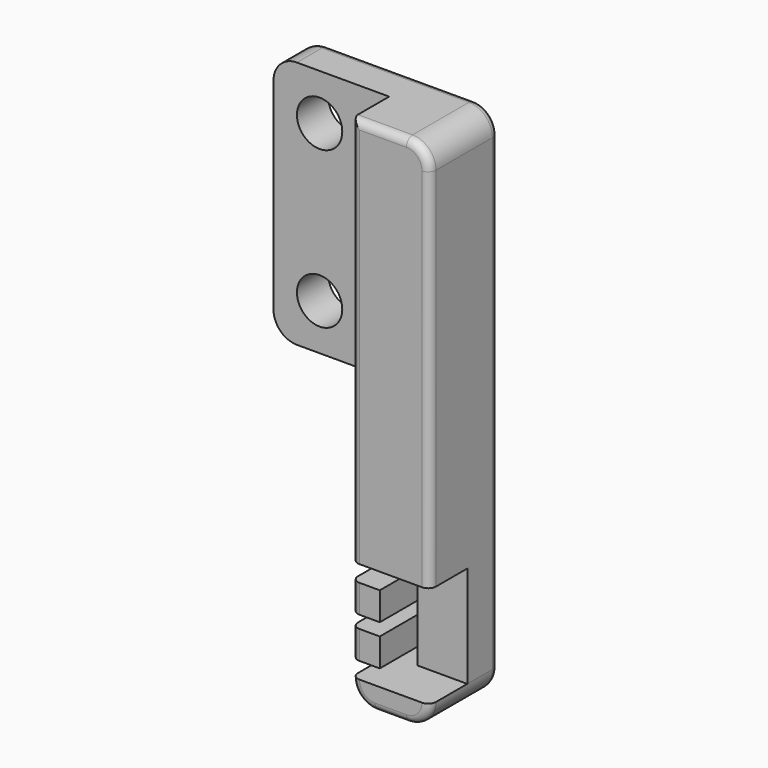
from build123d import *

# Parameters (mm, degrees)
F0_R        = 2.9
F0_W        = 10
F0_H        = 34.1
F1_DEPTH    = 5
F2_W        = 10
F2_H        = 3
F3_DEPTH    = 6
F4_W        = 3.6
F4_H        = 3.6
F5_DEPTH    = 6
F6_W        = 3.6
F6_H        = 2.1
F6_H_2      = 1.6
F7_DEPTH    = 5.001
F8_T1_DEPTH = 20
F8_T3_DEPTH = 26
F9_R        = 1


# Not quite as in the source:
# - a fillet or chamfer that OpenCascade refuses, or shapes differently, is made with other operations: its cross-section is extruded or revolved along the edge and cut away or added


with BuildPart() as f1:
    # F0 (on Front) → F1 (new body)
    with BuildSketch(Plane.XZ):
        Polygon((24.8, 0), (0, 0), (0, -31.8), (14.8, -31.8), (24.8, -31.8), align=None)
        with Locations((5.9, -25.9)):
            Circle(F0_R, mode=Mode.SUBTRACT)
        with Locations((5.9, -5.9)):
            Circle(F0_R, mode=Mode.SUBTRACT)
        with Locations((19.8, -48.85)):
            Rectangle(F0_W, F0_H)
    extrude(amount=F1_DEPTH)

    # F2 (on face) → F3 (join)
    with BuildSketch(Plane.XZ.offset(5)):
        Polygon((14.8, -49.9), (24.8, -49.9), (24.8, 0), (14.8, 0), (14.8, -31.8), align=None)
        with Locations((19.8, -64.4)):
            Rectangle(F2_W, F2_H)
    extrude(amount=F3_DEPTH)

    # F4 (on face) → F5 (join, through all)
    with BuildSketch(Plane.XZ.offset(5)):
        with Locations((16.6, -53.8)):
            Rectangle(F4_W, F4_H)
        with Locations((16.6, -59)):
            Rectangle(F4_W, F4_H)
    extrude(amount=F5_DEPTH)

    # F6 (on face) → F7 (cut, through all)
    with BuildSketch(Plane.XZ.offset(5)):
        with Locations((16.6, -50.95)):
            Rectangle(F6_W, F6_H)
        with Locations((16.6, -56.4)):
            Rectangle(F6_W, F6_H_2)
        with Locations((16.6, -61.85)):
            Rectangle(F6_W, F6_H)
    extrude(amount=-F7_DEPTH, mode=Mode.SUBTRACT)

    # F8: fillet of radius 3 on 5 edges, made by hand

    # F8_s2 → F8_t1 (cut)
    with BuildSketch(Plane.XZ.offset(-7.5)):
        with BuildLine():
            ThreePointArc((3, -31.8), (0.8786796564, -30.9213203436), (0, -28.8))
            Line((0, -28.8), (0, -31.8))
            Line((0, -31.8), (3, -31.8))
        make_face()
        with BuildLine():
            ThreePointArc((3, 0), (0.8786796564, -0.8786796564), (0, -3))
            Line((0, -3), (0, 0))
            Line((0, 0), (3, 0))
        make_face()
    extrude(amount=F8_T1_DEPTH, mode=Mode.SUBTRACT)

    # F8_s4 → F8_t3 (cut)
    with BuildSketch(Plane.XZ.offset(-7.5)):
        with BuildLine():
            ThreePointArc((21.8, 0), (23.9213203436, -0.8786796564), (24.8, -3))
            Line((24.8, -3), (24.8, 0))
            Line((24.8, 0), (21.8, 0))
        make_face()
        with BuildLine():
            ThreePointArc((21.8, -65.9), (23.9213203436, -65.0213203436), (24.8, -62.9))
            Line((24.8, -62.9), (24.8, -65.9))
            Line((24.8, -65.9), (21.8, -65.9))
        make_face()
        with BuildLine():
            ThreePointArc((14.8, -62.9), (15.6786796564, -65.0213203436), (17.8, -65.9))
            Line((17.8, -65.9), (14.8, -65.9))
            Line((14.8, -65.9), (14.8, -62.9))
        make_face()
    extrude(amount=F8_T3_DEPTH, mode=Mode.SUBTRACT)

    # F9
    f9_edges = [f1.edges().sort_by_distance(p)[0] for p in [
        (14.8, 0, -53.8),
        (14.8, 0, -59),
        (14.8, 0, -40.85),
        (24.8, -11, -26.45),
        (15.67868, 0, -65.02132),
        (14.8, -11, -24.95),
        (23.92132, -11, -65.02132),
        (12.4, 0, 0),
        (18.3, -11, 0),
        (23.92132, 0, -0.87868),
        (23.92132, -11, -0.87868),
        (8.9, 0, -31.8),
        (0.87868, 0, -30.92132),
        (0, 0, -15.9),
        (0.87868, 0, -0.87868),
        (24.8, 0, -32.95),
        (23.92132, 0, -65.02132),
        (19.8, 0, -65.9),
        (15.67868, -11, -65.02132),
        (14.8, -11, -59),
        (14.8, -11, -53.8),
        (19.8, -11, -65.9),
    ]]
    fillet(f9_edges, radius=F9_R)


solid = f1.part
